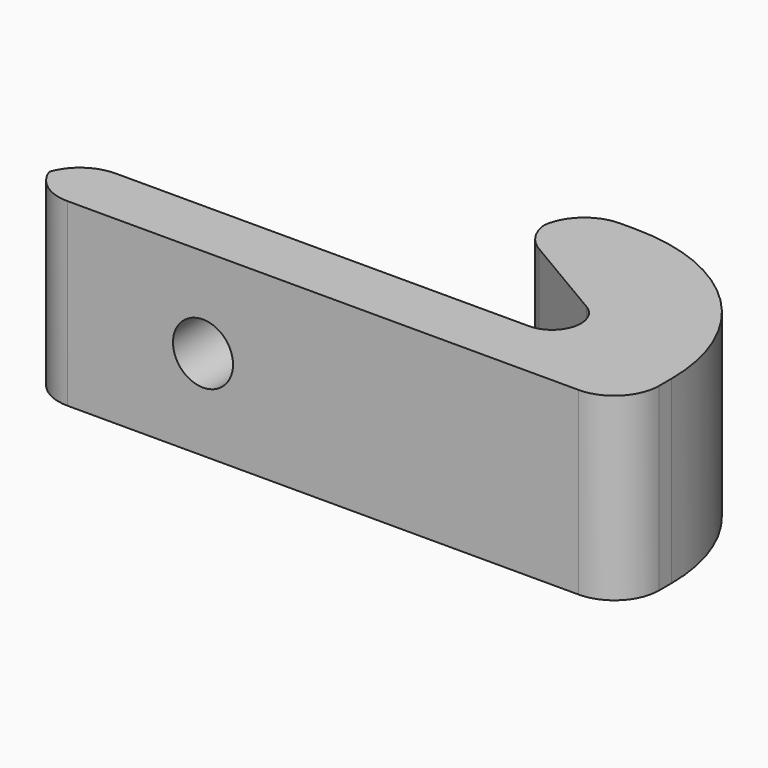
from build123d import *

# Parameters (mm, degrees)
F1_DEPTH    = 9.525
F2_R        = 1.5875
F3_DEPTH    = 12.701
F4_T1_DEPTH = 21.336
F4_T3_DEPTH = 16.266474116


# Not quite as in the source:
# - a fillet or chamfer that OpenCascade refuses, or shapes differently, is made with other operations: its cross-section is extruded or revolved along the edge and cut away or added


with BuildPart() as f1:
    # F0 (on Top) → F1 (new body)
    with BuildSketch(Plane.XY):
        with BuildLine():
            Line((24.2244322948, 0), (0, 0))
            Line((0, 0), (0, -3.175))
            Line((0, -3.175), (31.75, -3.175))
            Line((31.75, -3.175), (31.75, 0))
            Line((31.75, 0), (25.748250134, 1.5004374665))
            ThreePointArc((25.748250134, 1.5004374665), (25.2936999645, 0.4380706052), (24.2244322948, 0))
        make_face()
        with BuildLine():
            ThreePointArc((24.9994406757, 2.8362263561), (25.5538056385, 2.2692130656), (25.748250134, 1.5004374665))
            Line((25.748250134, 1.5004374665), (31.75, 0))
            ThreePointArc((31.75, 0), (28.9601920908, 6.7351920908), (22.225, 9.525))
            Line((22.225, 9.525), (19.05, 9.525))
            Line((19.05, 9.525), (19.05, 6.35))
            Line((19.05, 6.35), (24.9994406757, 2.8362263561))
        make_face()
    extrude(amount=F1_DEPTH)

    # F2 (on face) → F3 (cut, through all)
    with BuildSketch(Plane.XZ.offset(3.175)):
        with Locations((9.525, 4.7625)):
            Circle(F2_R)
    extrude(amount=-F3_DEPTH, mode=Mode.SUBTRACT)

    # F4: fillet of radius 2.3622 on 5 edges, made by hand

    # F4_s2 → F4_t1 (cut)
    with BuildSketch(Plane.XY.offset(-5.9055)):
        with BuildLine():
            ThreePointArc((29.3878, -3.175), (31.0581276385, -2.4831276385), (31.75, -0.8128))
            Line((31.75, -0.8128), (31.75, -3.175))
            Line((31.75, -3.175), (29.3878, -3.175))
        make_face()
        with BuildLine():
            ThreePointArc((21.4122, 9.525), (19.7418723615, 8.8331276385), (19.05, 7.1628))
            Line((19.05, 7.1628), (19.05, 9.525))
            Line((19.05, 9.525), (21.4122, 9.525))
        make_face()
        with BuildLine():
            ThreePointArc((0, -0.8128), (0.6918723615, -2.4831276385), (2.3622, -3.175))
            Line((2.3622, -3.175), (0, -3.175))
            Line((0, -3.175), (0, -0.8128))
        make_face()
        with BuildLine():
            ThreePointArc((2.3622, 0), (0.6918723615, -0.6918723615), (0, -2.3622))
            Line((0, -2.3622), (0, 0))
            Line((0, 0), (2.3622, 0))
        make_face()
    extrude(amount=F4_T1_DEPTH, mode=Mode.SUBTRACT)

    # F4_s4 → F4_t3 (cut)
    with BuildSketch(Plane.XY.offset(-3.370737058)):
        with BuildLine():
            ThreePointArc((20.2109370097, 5.6643439713), (19.3606624942, 6.5273197158), (19.05, 7.6982948232))
            Line((19.05, 7.6982948232), (19.05, 6.35))
            Line((19.05, 6.35), (20.2109370097, 5.6643439713))
        make_face()
    extrude(amount=F4_T3_DEPTH, mode=Mode.SUBTRACT)


solid = f1.part
